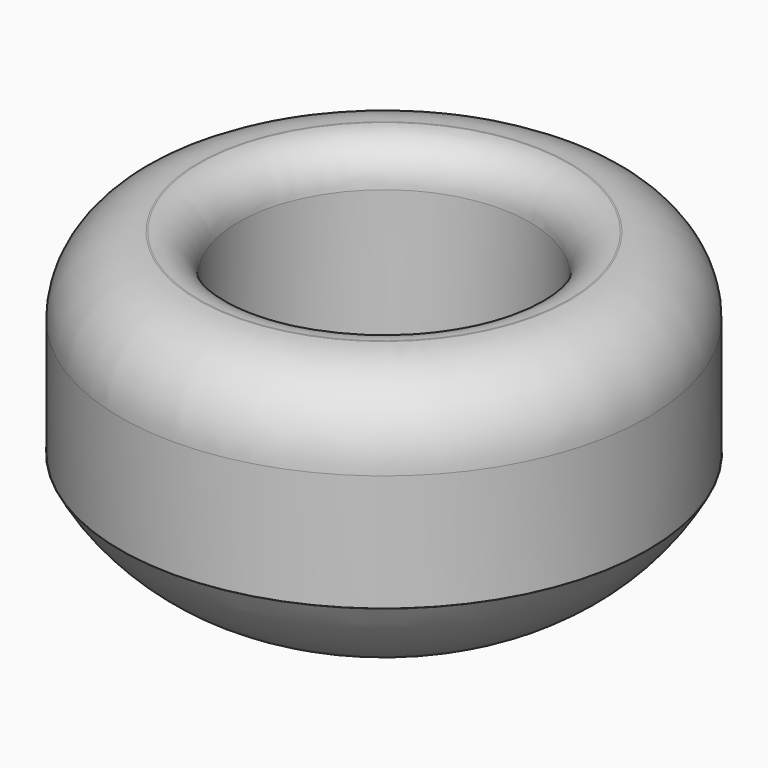
from build123d import *

# Parameters (mm, degrees)
F0_R     = 33.8982818127
F0_R_2   = 18.7267733827
F1_DEPTH = 40
F2_R     = 33.9321571181
F3_DEPTH = 15
F4_R     = 10
F5_R     = 5


# Not quite as in the source:
# - a fillet or chamfer that OpenCascade refuses, or shapes differently, is made with other operations: its cross-section is extruded or revolved along the edge and cut away or added


with BuildPart() as f1:
    # F0 (on Top) → F1 (new body)
    with BuildSketch(Plane.XY):
        Circle(F0_R)
        Circle(F0_R_2, mode=Mode.SUBTRACT)
    extrude(amount=F1_DEPTH)

    # F2 (on Top) → F3 (join)
    with BuildSketch(Plane.XY):
        Circle(F2_R)
    extrude(amount=F3_DEPTH)

    # F4
    f4_edges = [f1.edges().sort_by_distance(p)[0] for p in [
        (-33.898282, 0, 40),
    ]]
    fillet(f4_edges, radius=F4_R)

    # F5
    f5_edges = [f1.edges().sort_by_distance(p)[0] for p in [
        (-18.726773, 0, 40),
    ]]
    fillet(f5_edges, radius=F5_R)

    # F6: fillet of radius 28.7291413922 on 1 edges, made by hand

    # F6_s1 → F6_t2 (revolve, cut)
    with BuildSketch(Plane.XZ):
        with BuildLine():
            ThreePointArc((33.9321571181, 15), (23.3746370554, 4.0330889811), (8.6957896741, 0))
            Line((8.6957896741, 0), (33.9321571181, 0))
            Line((33.9321571181, 0), (33.9321571181, 15))
        make_face()
    revolve(axis=Axis((0, 0, 0), (0, 0, 1)), mode=Mode.SUBTRACT)


solid = f1.part
